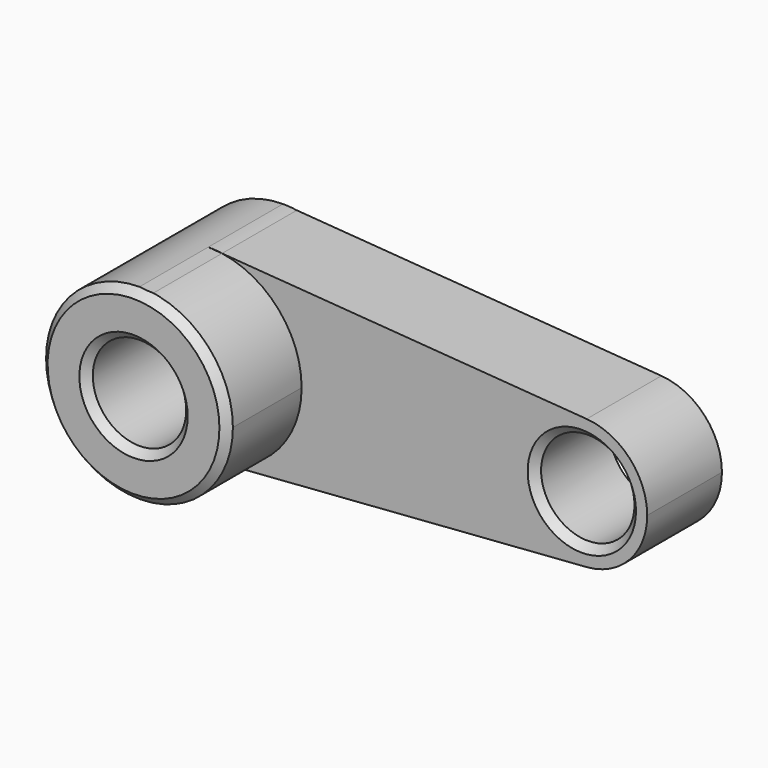
from build123d import *

# Parameters (mm, degrees)
F0_R        = 12.5
F1_DEPTH    = 25
F2_DEPTH    = 50
F3_T4_ANGLE = 203.6133668192
F3_T6_ANGLE = 179.9906971182


# Not quite as in the source:
# - a fillet or chamfer that OpenCascade refuses, or shapes differently, is made with other operations: its cross-section is extruded or revolved along the edge and cut away or added


with BuildPart() as f1:
    # F0 (on Front) → F1 (new body)
    with BuildSketch(Plane.XZ):
        with BuildLine():
            Line((3.7051688109, 24.7239099675), (0, 25))
            ThreePointArc((0, 25), (-25, 0), (0, -25))
            Line((0, -25), (3.7051688109, -24.7239099675))
            ThreePointArc((3.7051688109, -24.7239099675), (18.9424024383, -16.3151889313), (25, 0))
            ThreePointArc((25, 0), (18.9424024383, 16.3151889313), (3.7051688109, 24.7239099675))
        make_face()
        Circle(F0_R, mode=Mode.SUBTRACT)
        with BuildLine():
            ThreePointArc((3.7051688109, 24.7239099675), (1.8577204864, 24.9308819458), (0, 25))
            Line((0, 25), (3.7051688109, 24.7239099675))
        make_face()
        with BuildLine():
            Line((3.7051688109, -24.7239099675), (0, -25))
            ThreePointArc((0, -25), (1.8577204864, -24.9308819458), (3.7051688109, -24.7239099675))
        make_face()
        with BuildLine():
            Line((101.3004043405, 17.451617362), (3.7051688109, 24.7239099675))
            ThreePointArc((3.7051688109, 24.7239099675), (18.9424024383, 16.3151889313), (25, 0))
            ThreePointArc((25, 0), (18.9424024383, -16.3151889313), (3.7051688109, -24.7239099675))
            Line((3.7051688109, -24.7239099675), (101.3004043405, -17.451617362))
            ThreePointArc((101.3004043405, -17.451617362), (82.5, 0), (101.3004043405, 17.451617362))
        make_face()
        with BuildLine():
            ThreePointArc((117.5, 0), (112.8258932624, 11.9057323177), (101.3004043405, 17.451617362))
            ThreePointArc((101.3004043405, 17.451617362), (82.5, 0), (101.3004043405, -17.451617362))
            ThreePointArc((101.3004043405, -17.451617362), (112.8258932624, -11.9057323177), (117.5, 0))
        make_face()
        with Locations((100, 0)):
            Circle(F0_R, mode=Mode.SUBTRACT)
    extrude(amount=F1_DEPTH)

    # F0 (on Front) → F2 (join)
    with BuildSketch(Plane.XZ):
        with BuildLine():
            Line((3.7051688109, 24.7239099675), (0, 25))
            ThreePointArc((0, 25), (-25, 0), (0, -25))
            Line((0, -25), (3.7051688109, -24.7239099675))
            ThreePointArc((3.7051688109, -24.7239099675), (18.9424024383, -16.3151889313), (25, 0))
            ThreePointArc((25, 0), (18.9424024383, 16.3151889313), (3.7051688109, 24.7239099675))
        make_face()
        Circle(F0_R, mode=Mode.SUBTRACT)
    extrude(amount=F2_DEPTH)

    # F3: chamfer of 2 on 4 edges, made by hand

    # F3_s1 → F3_t2 (revolve, cut)
    with BuildSketch(Plane.XY):
        Polygon((14.5, -50), (12.5, -48), (12.5, -50), align=None)
    revolve(axis=Axis((0, -50, 0), (0, -1, 0)), mode=Mode.SUBTRACT)

    # F3_s3 → F3_t4 (revolve, cut)
    with BuildSketch(Plane(origin=(0, 0, 0), x_dir=(0, 1, 0), z_dir=(0.9788435281, 0, -0.2046102329))):
        Polygon((-48, 25), (-50, 23), (-50, 25), align=None)
    revolve(axis=Axis((0, -50, 0), (0, -1, 0)), revolution_arc=F3_T4_ANGLE, mode=Mode.SUBTRACT)

    # F3_s5 → F3_t6 (revolve, cut)
    with BuildSketch(Plane(origin=(0, 0, 0), x_dir=(0, 1, 0), z_dir=(-0.9999999967, 0, 8.1183e-05))):
        Polygon((-48, -25), (-50, -23), (-50, -25), align=None)
    revolve(axis=Axis((0, -50, 0), (0, 1, 0)), revolution_arc=F3_T6_ANGLE, mode=Mode.SUBTRACT)

    # F3_s7 → F3_t8 (revolve, cut)
    with BuildSketch(Plane.XY):
        Polygon((114.5, -25), (112.5, -23), (112.5, -25), align=None)
    revolve(axis=Axis((100, -25, 0), (0, -1, 0)), mode=Mode.SUBTRACT)


solid = f1.part
